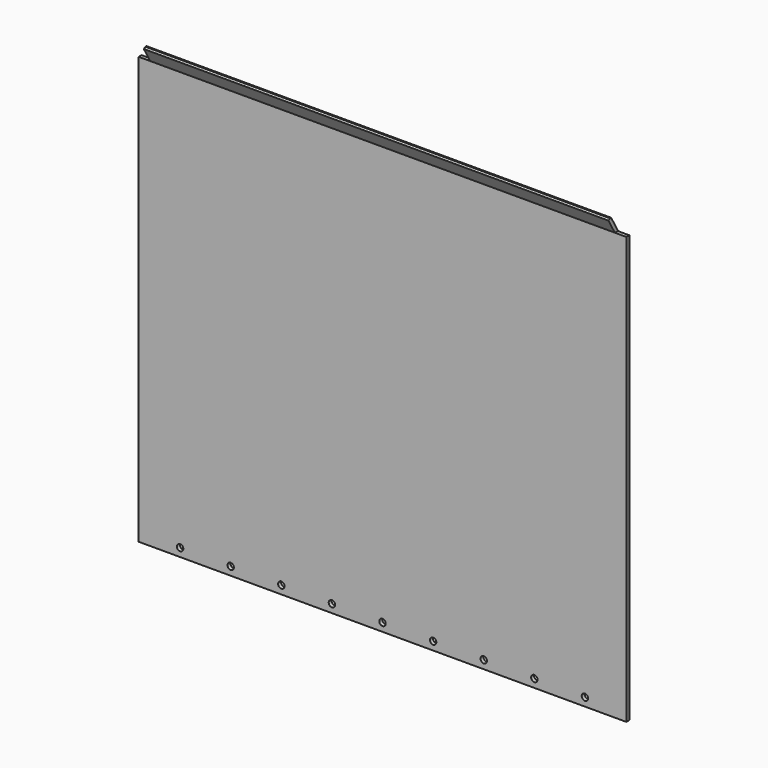
from build123d import *

# Parameters (mm, degrees)
F1_DEPTH = 530
F3_DEPTH = 25
F4_R     = 7
F5_DEPTH = 5.001
F7_DEPTH = 1060.001
F8_DEPTH = 3


# Not quite as in the source:
# - a pattern or mirror of a feature is missing from the dataset's text; its kind, count and spacing are read off the source's solid


with BuildPart() as f1:
    # F0 (on Right) → F1 (new body, symmetric)
    with BuildSketch(Plane.YZ):
        Polygon((0, 940), (0, 0), (-6.4704761276, -24.1481456572), (-1.6408469961, -25.4422408827), (5, -0.6582624879), (5, 941.3397459622), (-13.1698729811, 972.8108891325), (-17.5, 970.3108891325), align=None)
    extrude(amount=F1_DEPTH, both=True)

    # F2 (on face) → F3 (cut)
    with BuildSketch(Plane.YZ.offset(530)):
        Polygon((5, 0), (0, 0), (-6.4704761276, -24.1481456572), (-1.6408469961, -25.4422408827), (5, -0.6582624879), align=None)
        Polygon((-17.5, 970.3108891325), (0, 940), (5, 940), (5, 941.3397459622), (-13.1698729811, 972.8108891325), align=None)
    f3 = extrude(amount=-F3_DEPTH, mode=Mode.SUBTRACT)

    # F3_copies: F3 across plane
    add(f3.mirror(Plane(origin=(0, 0, 0), x_dir=(0, 0, -1), z_dir=(-1, 0, 0))), mode=Mode.SUBTRACT)

    # F4 (on face) → F5 (cut, through all)
    with BuildSketch(Plane.XZ):
        with Locations((0, 30)):
            Circle(F4_R)
        with Locations((110, 30)):
            Circle(F4_R)
        with Locations((220, 30)):
            Circle(F4_R)
        with Locations((330, 30)):
            Circle(F4_R)
        with Locations((440, 30)):
            Circle(F4_R)
        with Locations((-110, 30)):
            Circle(F4_R)
        with Locations((-220, 30)):
            Circle(F4_R)
        with Locations((-330, 30)):
            Circle(F4_R)
        with Locations((-440, 30)):
            Circle(F4_R)
    extrude(amount=-F5_DEPTH, mode=Mode.SUBTRACT)

    # F6 (on face) → F7 (cut, through all)
    with BuildSketch(Plane.YZ.offset(530)):
        Polygon((0, 12), (0, 0), (-6.4704761276, -24.1481456572), (-1.6408469961, -25.4422408827), (5, -0.6582624879), (5, 12), align=None)
    extrude(amount=-F7_DEPTH, mode=Mode.SUBTRACT)

    # F8 (add): faces of the model
    f8_faces = [f1.faces().sort_by_distance(p)[0] for p in [
        (0, 5, 477.2673971314),
        (0, -4.0849364905, 957.0753175473),
    ]]
    extrude(f8_faces, amount=F8_DEPTH, dir=(0, 1, 0))


solid = f1.part
